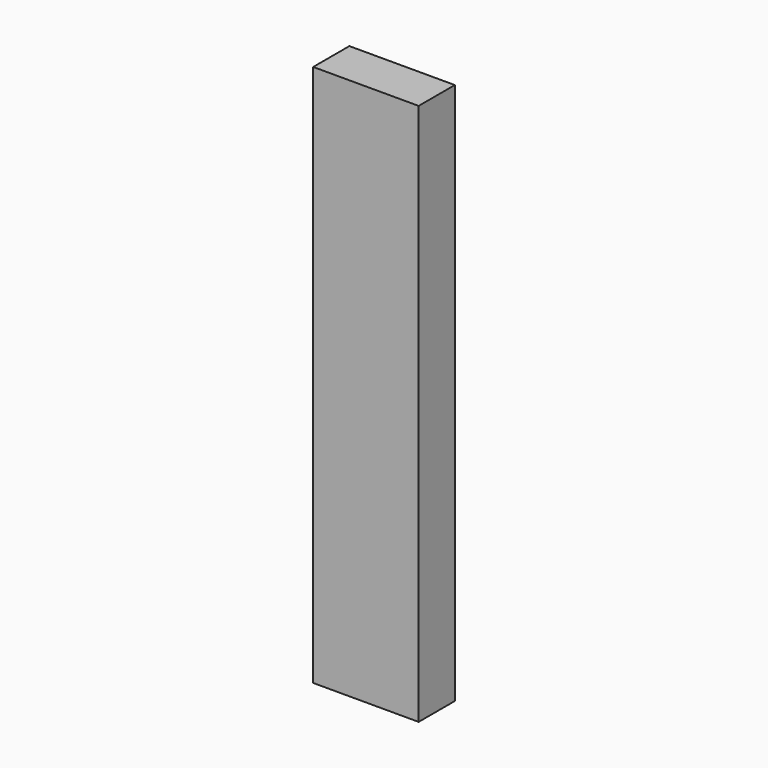
from build123d import *

# Parameters (mm, degrees)
F0_W     = 88.9
F0_H     = 457.2
F1_DEPTH = 38.1


with BuildPart() as f1:
    # F0 (on Front) → F1 (new body)
    with BuildSketch(Plane.XZ):
        with Locations((44.45, 228.6)):
            Rectangle(F0_W, F0_H)
    extrude(amount=-F1_DEPTH)


solid = f1.part
